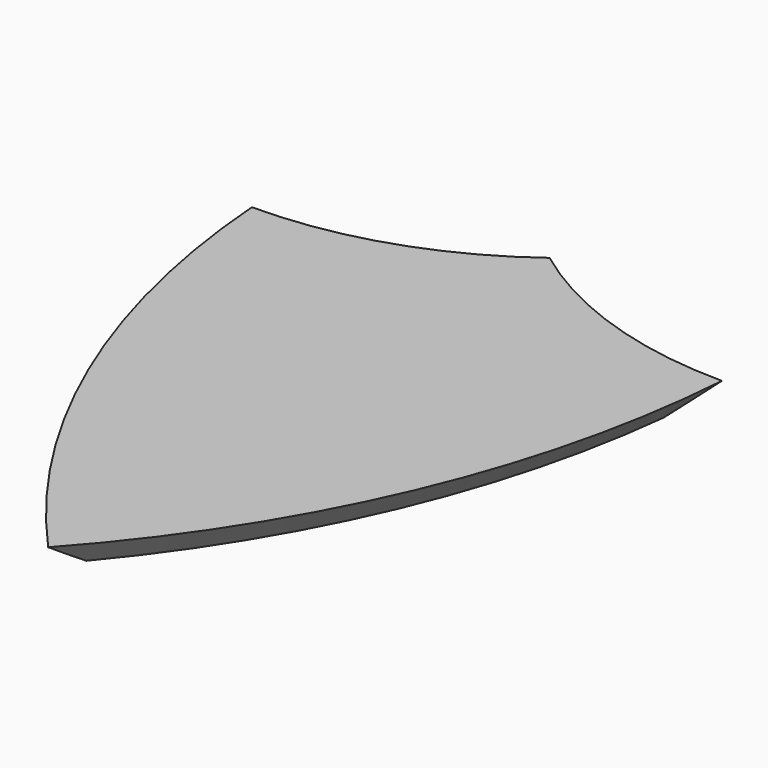
from build123d import *

# Parameters (mm, degrees)
F1_DEPTH = 2.54
F2_SIZE  = 2.53999


# Not quite as in the source:
# - a fillet or chamfer is up to 0.001 mm smaller than in the source, because OpenCascade refuses the exact size


with BuildPart() as f1:
    # F0 (on Top) → F1 (new body)
    with BuildSketch(Plane.XY):
        with BuildLine():
            ThreePointArc((0, 25.4), (-9.009768429, 20.6793052869), (-19.05, 19.05))
            ThreePointArc((-19.05, 19.05), (-13.2442322719, -4.768956688), (0, -25.4))
            ThreePointArc((0, -25.4), (13.2442322719, -4.768956688), (19.05, 19.05))
            ThreePointArc((19.05, 19.05), (9.009768429, 20.6793052869), (0, 25.4))
        make_face()
    extrude(amount=F1_DEPTH)

    # F2 (size 2.54 in the source; OpenCascade refuses exactly that, so slightly less here)
    f2_edges = [f1.edges().sort_by_distance(p)[0] for p in [
        (13.244232, -4.768957, 0),
        (-13.244232, -4.768957, 0),
        (-9.009768, 20.679305, 0),
        (9.009768, 20.679305, 0),
    ]]
    chamfer(f2_edges, length=F2_SIZE)


solid = f1.part
